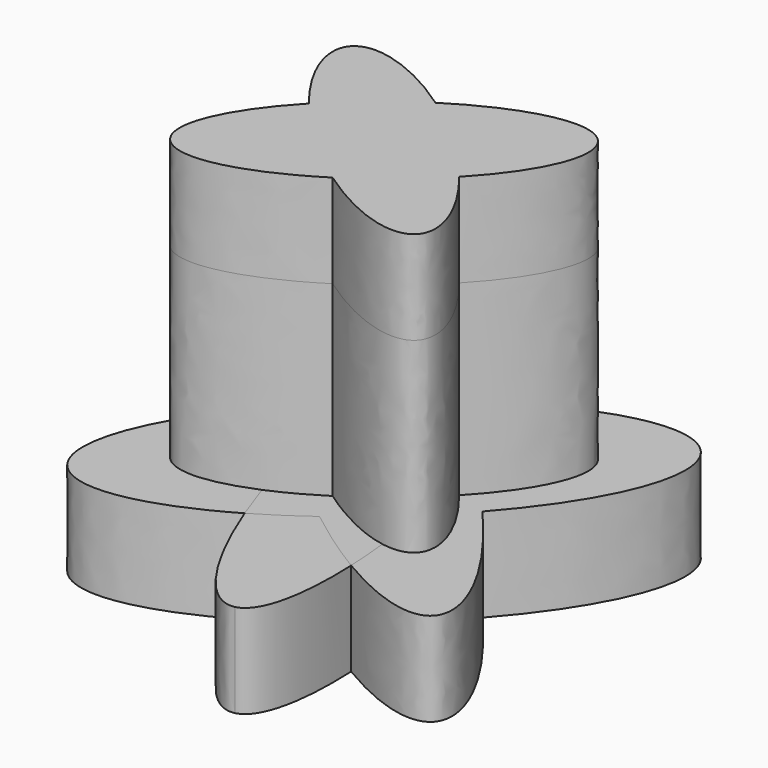
from build123d import *

# Parameters (mm, degrees)
F1_DEPTH = 25.4
F3_DEPTH = 25.4
F4_DEPTH = 76.2
F5_DEPTH = 25.4
F7_DEPTH = 25.4


with BuildPart() as f1:
    # F0 (on Top) → F1 (new body)
    with BuildSketch(Plane.XY):
        with BuildLine():
            add(Edge.make_bspline(
                [(31.4708654555, -5.9622764169), (63.3714591709, 30.0253372008), (50.3187514842, 44.7141192853)],
                knots=[5.0072825933, 5.0072825933, 5.0072825933, 6.2831853072, 6.2831853072, 6.2831853072], degree=2, weights=[1, 0.8033175142, 1]))
            add(Edge.make_bspline(
                [(50.3187514842, 44.7141192853), (36.2964379825, 60.4940411444), (-5.9006929596, 29.3159511373)],
                knots=[0, 0, 0, 1.3451277265, 1.3451277265, 1.3451277265], degree=2, weights=[1, 0.7822269683, 1]))
            add(Edge.make_bspline(
                [(31.4708654555, -5.9622764169), (14.5963553051, 13.331100287), (-5.9006929596, 29.3159511373)],
                knots=[4.3323479681, 4.3323479681, 4.3323479681, 5.0523278478, 5.0523278478, 5.0523278478], degree=2, weights=[1, 0.9359003676, 1]))
        make_face()
        with BuildLine():
            add(Edge.make_bspline(
                [(31.4708654555, -5.9622764169), (14.5963553051, 13.331100287), (-5.9006929596, 29.3159511373)],
                knots=[4.3323479681, 4.3323479681, 4.3323479681, 5.0523278478, 5.0523278478, 5.0523278478], degree=2, weights=[1, 0.9359003676, 1]))
            add(Edge.make_bspline(
                [(-5.9006929596, 29.3159511373), (-20.0111187013, 18.8902156907), (-31.4708654555, 5.9622764169)],
                knots=[1.3451277265, 1.3451277265, 1.3451277265, 1.8656899397, 1.8656899397, 1.8656899397], degree=2, weights=[1, 0.9663176729, 1]))
            add(Edge.make_bspline(
                [(-31.4708654555, 5.9622764169), (-14.5963553051, -13.331100287), (5.9006929596, -29.3159511373)],
                knots=[1.1907553145, 1.1907553145, 1.1907553145, 1.9107351942, 1.9107351942, 1.9107351942], degree=2, weights=[1, 0.9359003676, 1]))
            add(Edge.make_bspline(
                [(5.9006929596, -29.3159511373), (20.0111187013, -18.8902156907), (31.4708654555, -5.9622764169)],
                knots=[4.4867203801, 4.4867203801, 4.4867203801, 5.0072825933, 5.0072825933, 5.0072825933], degree=2, weights=[1, 0.9663176729, 1]))
        make_face()
        with BuildLine():
            add(Edge.make_bspline(
                [(-5.9006929596, 29.3159511373), (-20.0111187013, 18.8902156907), (-31.4708654555, 5.9622764169)],
                knots=[1.3451277265, 1.3451277265, 1.3451277265, 1.8656899397, 1.8656899397, 1.8656899397], degree=2, weights=[1, 0.9663176729, 1]))
            add(Edge.make_bspline(
                [(-5.9006929596, 29.3159511373), (-44.4032618327, 59.3426073095), (-53.3079244196, 49.8132295907)],
                knots=[5.0523278478, 5.0523278478, 5.0523278478, 6.2831853072, 6.2831853072, 6.2831853072], degree=2, weights=[1, 0.8165260126, 1]))
            add(Edge.make_bspline(
                [(-53.3079244196, 49.8132295907), (-61.8390610835, 40.6835828637), (-31.4708654555, 5.9622764169)],
                knots=[0, 0, 0, 1.1907553145, 1.1907553145, 1.1907553145], degree=2, weights=[1, 0.8279367596, 1]))
        make_face()
        with BuildLine():
            add(Edge.make_bspline(
                [(5.9006929596, -29.3159511373), (150.5818649005, -142.1471707573), (31.4708654555, -5.9622764169)],
                knots=[1.9107351942, 1.9107351942, 1.9107351942, 4.3323479681, 4.3323479681, 4.3323479681], degree=2, weights=[1, 0.352264818, 1]))
            add(Edge.make_bspline(
                [(5.9006929596, -29.3159511373), (20.0111187013, -18.8902156907), (31.4708654555, -5.9622764169)],
                knots=[4.4867203801, 4.4867203801, 4.4867203801, 5.0072825933, 5.0072825933, 5.0072825933], degree=2, weights=[1, 0.9663176729, 1]))
        make_face()
        with BuildLine():
            add(Edge.make_bspline(
                [(-31.4708654555, 5.9622764169), (-14.5963553051, -13.331100287), (5.9006929596, -29.3159511373)],
                knots=[1.1907553145, 1.1907553145, 1.1907553145, 1.9107351942, 1.9107351942, 1.9107351942], degree=2, weights=[1, 0.9359003676, 1]))
            add(Edge.make_bspline(
                [(-31.4708654555, 5.9622764169), (-64.5405485612, -31.3442072393), (-49.679335289, -45.3729843571), (-34.8181220167, -59.4017614749), (5.9006929596, -29.3159511373)],
                knots=[1.8656899397, 1.8656899397, 1.8656899397, 3.1762051599, 3.1762051599, 4.4867203801, 4.4867203801, 4.4867203801], degree=2, weights=[1, 0.7928909762, 1, 0.7928909762, 1]))
        make_face()
    extrude(amount=F1_DEPTH)

    # F2 (on Top) → F3 (join)
    with BuildSketch(Plane.XY):
        with BuildLine():
            add(Edge.make_bspline(
                [(22.9789679263, -3.1803961662), (12.2875146744, 10.0941238239), (-2.2086285063, 20.2431125515)],
                knots=[1.1162608862, 1.1162608862, 1.1162608862, 1.9250688609, 1.9250688609, 1.9250688609], degree=2, weights=[1, 0.9193370741, 1]))
            add(Edge.make_bspline(
                [(22.9789679263, -3.1803961662), (118.1418333631, 97.0528480616), (-2.2086285063, 20.2431125515)],
                knots=[1.9344756774, 1.9344756774, 1.9344756774, 4.4740450435, 4.4740450435, 4.4740450435], degree=2, weights=[1, 0.2964865155, 1]))
        make_face()
        with BuildLine():
            add(Edge.make_bspline(
                [(-22.9789679263, 3.1803961662), (-12.2875146744, -10.0941238239), (2.2086285063, -20.2431125515)],
                knots=[4.2578535397, 4.2578535397, 4.2578535397, 5.0666615145, 5.0666615145, 5.0666615145], degree=2, weights=[1, 0.9193370741, 1]))
            add(Edge.make_bspline(
                [(2.2086285063, -20.2431125515), (13.8075396903, -12.8404878636), (22.9789679263, -3.1803961662)],
                knots=[1.33245239, 1.33245239, 1.33245239, 1.9344756774, 1.9344756774, 1.9344756774], degree=2, weights=[1, 0.9550370392, 1]))
            add(Edge.make_bspline(
                [(22.9789679263, -3.1803961662), (12.2875146744, 10.0941238239), (-2.2086285063, 20.2431125515)],
                knots=[1.1162608862, 1.1162608862, 1.1162608862, 1.9250688609, 1.9250688609, 1.9250688609], degree=2, weights=[1, 0.9193370741, 1]))
            add(Edge.make_bspline(
                [(-2.2086285063, 20.2431125515), (-13.8075396903, 12.8404878636), (-22.9789679263, 3.1803961662)],
                knots=[4.4740450435, 4.4740450435, 4.4740450435, 5.076068331, 5.076068331, 5.076068331], degree=2, weights=[1, 0.9550370392, 1]))
        make_face()
        with BuildLine():
            add(Edge.make_bspline(
                [(-22.9789679263, 3.1803961662), (-43.34502165, -18.2707825838), (-35.7845425606, -27.9503762722)],
                knots=[5.076068331, 5.076068331, 5.076068331, 6.2831853072, 6.2831853072, 6.2831853072], degree=2, weights=[1, 0.8233211201, 1]))
            add(Edge.make_bspline(
                [(-35.7845425606, -27.9503762722), (-27.1629197213, -38.988539996), (2.2086285063, -20.2431125515)],
                knots=[0, 0, 0, 1.33245239, 1.33245239, 1.33245239], degree=2, weights=[1, 0.7861595589, 1]))
            add(Edge.make_bspline(
                [(-22.9789679263, 3.1803961662), (-12.2875146744, -10.0941238239), (2.2086285063, -20.2431125515)],
                knots=[4.2578535397, 4.2578535397, 4.2578535397, 5.0666615145, 5.0666615145, 5.0666615145], degree=2, weights=[1, 0.9193370741, 1]))
        make_face()
        with BuildLine():
            add(Edge.make_bspline(
                [(-2.2086285063, 20.2431125515), (-81.3451205129, 75.6478747217), (-22.9789679263, 3.1803961662)],
                knots=[1.9250688609, 1.9250688609, 1.9250688609, 4.2578535397, 4.2578535397, 4.2578535397], degree=2, weights=[1, 0.3934708938, 1]))
            add(Edge.make_bspline(
                [(-2.2086285063, 20.2431125515), (-13.8075396903, 12.8404878636), (-22.9789679263, 3.1803961662)],
                knots=[4.4740450435, 4.4740450435, 4.4740450435, 5.076068331, 5.076068331, 5.076068331], degree=2, weights=[1, 0.9550370392, 1]))
        make_face()
    extrude(amount=F3_DEPTH)

    # F2 (on Top) → F4 (join)
    with BuildSketch(Plane.XY):
        with BuildLine():
            add(Edge.make_bspline(
                [(-22.9789679263, 3.1803961662), (-43.34502165, -18.2707825838), (-35.7845425606, -27.9503762722)],
                knots=[5.076068331, 5.076068331, 5.076068331, 6.2831853072, 6.2831853072, 6.2831853072], degree=2, weights=[1, 0.8233211201, 1]))
            add(Edge.make_bspline(
                [(-35.7845425606, -27.9503762722), (-27.1629197213, -38.988539996), (2.2086285063, -20.2431125515)],
                knots=[0, 0, 0, 1.33245239, 1.33245239, 1.33245239], degree=2, weights=[1, 0.7861595589, 1]))
            add(Edge.make_bspline(
                [(-22.9789679263, 3.1803961662), (-12.2875146744, -10.0941238239), (2.2086285063, -20.2431125515)],
                knots=[4.2578535397, 4.2578535397, 4.2578535397, 5.0666615145, 5.0666615145, 5.0666615145], degree=2, weights=[1, 0.9193370741, 1]))
        make_face()
        with BuildLine():
            add(Edge.make_bspline(
                [(-22.9789679263, 3.1803961662), (-12.2875146744, -10.0941238239), (2.2086285063, -20.2431125515)],
                knots=[4.2578535397, 4.2578535397, 4.2578535397, 5.0666615145, 5.0666615145, 5.0666615145], degree=2, weights=[1, 0.9193370741, 1]))
            add(Edge.make_bspline(
                [(2.2086285063, -20.2431125515), (13.8075396903, -12.8404878636), (22.9789679263, -3.1803961662)],
                knots=[1.33245239, 1.33245239, 1.33245239, 1.9344756774, 1.9344756774, 1.9344756774], degree=2, weights=[1, 0.9550370392, 1]))
            add(Edge.make_bspline(
                [(22.9789679263, -3.1803961662), (12.2875146744, 10.0941238239), (-2.2086285063, 20.2431125515)],
                knots=[1.1162608862, 1.1162608862, 1.1162608862, 1.9250688609, 1.9250688609, 1.9250688609], degree=2, weights=[1, 0.9193370741, 1]))
            add(Edge.make_bspline(
                [(-2.2086285063, 20.2431125515), (-13.8075396903, 12.8404878636), (-22.9789679263, 3.1803961662)],
                knots=[4.4740450435, 4.4740450435, 4.4740450435, 5.076068331, 5.076068331, 5.076068331], degree=2, weights=[1, 0.9550370392, 1]))
        make_face()
        with BuildLine():
            add(Edge.make_bspline(
                [(2.2086285063, -20.2431125515), (13.8075396903, -12.8404878636), (22.9789679263, -3.1803961662)],
                knots=[1.33245239, 1.33245239, 1.33245239, 1.9344756774, 1.9344756774, 1.9344756774], degree=2, weights=[1, 0.9550370392, 1]))
            add(Edge.make_bspline(
                [(2.2086285063, -20.2431125515), (25.793459334, -36.7552412762), (32.5327925384, -29.2628221214)],
                knots=[5.0666615145, 5.0666615145, 5.0666615145, 6.2831853072, 6.2831853072, 6.2831853072], degree=2, weights=[1, 0.8206424823, 1]))
            add(Edge.make_bspline(
                [(32.5327925384, -29.2628221214), (38.5754174401, -22.5449648519), (22.9789679263, -3.1803961662)],
                knots=[0, 0, 0, 1.1162608862, 1.1162608862, 1.1162608862], degree=2, weights=[1, 0.8482467126, 1]))
        make_face()
        with BuildLine():
            add(Edge.make_bspline(
                [(-2.2086285063, 20.2431125515), (-81.3451205129, 75.6478747217), (-22.9789679263, 3.1803961662)],
                knots=[1.9250688609, 1.9250688609, 1.9250688609, 4.2578535397, 4.2578535397, 4.2578535397], degree=2, weights=[1, 0.3934708938, 1]))
            add(Edge.make_bspline(
                [(-2.2086285063, 20.2431125515), (-13.8075396903, 12.8404878636), (-22.9789679263, 3.1803961662)],
                knots=[4.4740450435, 4.4740450435, 4.4740450435, 5.076068331, 5.076068331, 5.076068331], degree=2, weights=[1, 0.9550370392, 1]))
        make_face()
        with BuildLine():
            add(Edge.make_bspline(
                [(22.9789679263, -3.1803961662), (12.2875146744, 10.0941238239), (-2.2086285063, 20.2431125515)],
                knots=[1.1162608862, 1.1162608862, 1.1162608862, 1.9250688609, 1.9250688609, 1.9250688609], degree=2, weights=[1, 0.9193370741, 1]))
            add(Edge.make_bspline(
                [(22.9789679263, -3.1803961662), (118.1418333631, 97.0528480616), (-2.2086285063, 20.2431125515)],
                knots=[1.9344756774, 1.9344756774, 1.9344756774, 4.4740450435, 4.4740450435, 4.4740450435], degree=2, weights=[1, 0.2964865155, 1]))
        make_face()
    extrude(amount=F4_DEPTH)

    # F5 (add): a face of the model
    f5_faces = [f1.faces().sort_by_distance(p)[0] for p in [
        (0.0001411459, 0.0005968087, 76.2),
    ]]
    extrude(f5_faces, amount=F5_DEPTH)

    # F6 (on Top) → F7 (join)
    with BuildSketch(Plane.XY):
        with BuildLine():
            add(Edge.make_bspline(
                [(17.9541409016, -72.9985460639), (48.9716433746, -65.3697282334), (6.5316807857, 40.3136819472), (-35.9082818031, 145.9970921278), (-24.4858216873, 32.6848641167), (-13.0633615715, -80.6273638944), (17.9541409016, -72.9985460639)],
                knots=[0, 0, 0, 2.0943951024, 2.0943951024, 4.1887902048, 4.1887902048, 6.2831853072, 6.2831853072, 6.2831853072], degree=2, weights=[1, 0.5, 1, 0.5, 1, 0.5, 1]))
        make_face()
    extrude(amount=F7_DEPTH)


solid = f1.part
